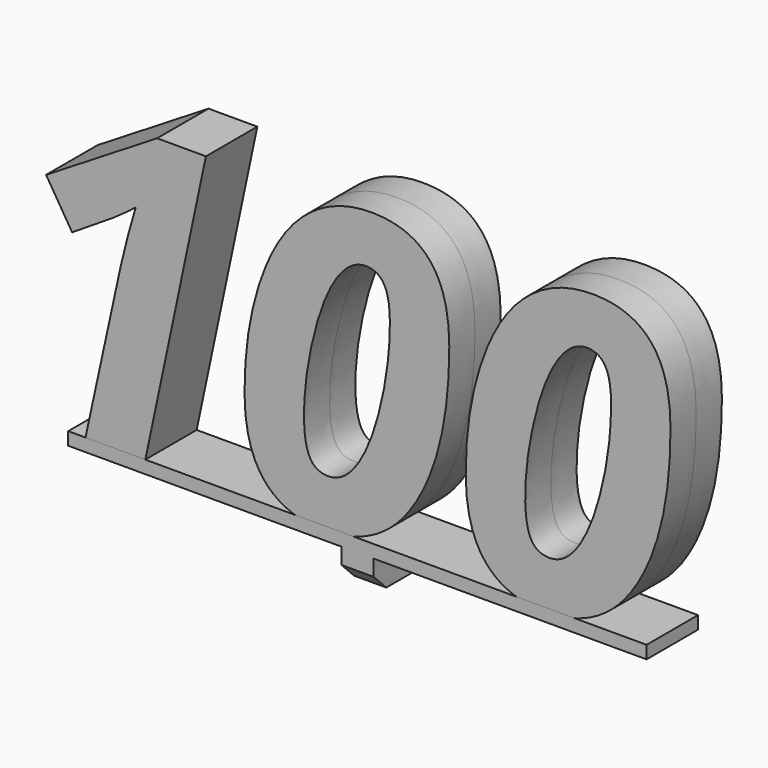
from build123d import *

# Parameters (mm, degrees)
F0_TEXT_SIZE = 62.5
F1_DEPTH     = 5
F2_W         = 90
F2_H         = 10
F3_DEPTH     = 2
F4_W         = 5
F4_H         = 10
F5_DEPTH     = 5
F6_SIZE      = 2.5


# Not quite as in the source:
# - Text() gives the source's letters only with a copy of the font that has no kerning and outlines rounded to 1/6400 em; it was checked with that copy


with BuildPart() as f1:
    # F0 (on Front) → F1 (new body, symmetric)
    with BuildSketch(Plane.XZ):
        with Locations((-54.0000047238, 0)):
            Text('100', F0_TEXT_SIZE, font='Open Sans', font_style=FontStyle.BOLDITALIC, text_align=(TextAlign.LEFT, TextAlign.BOTTOM))
    extrude(amount=F1_DEPTH, both=True)


with BuildPart() as f3:
    # F2 (on Top) → F3 (new body)
    with BuildSketch(Plane.XY):
        Rectangle(F2_W, F2_H)
    extrude(amount=-F3_DEPTH)

    # F4 (on face) → F5 (join)
    with BuildSketch(Plane(origin=(0, 0, -2), x_dir=(1, 0, 0), z_dir=(0, 0, -1))):
        Rectangle(F4_W, F4_H)
    extrude(amount=F5_DEPTH)

    # F6
    f6_edges = [f3.edges().sort_by_distance(p)[0] for p in [
        (0, -5, -7),
        (0, 5, -7),
    ]]
    chamfer(f6_edges, length=F6_SIZE)


solid = Compound([f1.part, f3.part])
